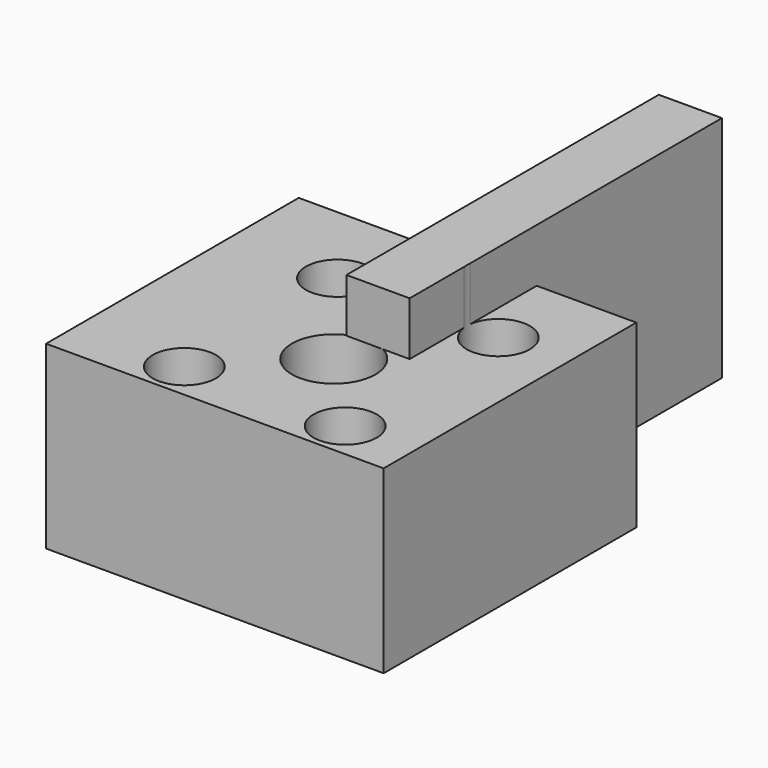
from build123d import *

# Parameters (mm, degrees)
F0_W     = 156.9848433137
F0_H     = 92.025604099
F1_DEPTH = 25.4
F2_W     = 135.7623711228
F2_H     = 72.5497286767
F4_DEPTH = 127
F6_D     = 25.4
F8_R     = 16.8146432666
F9_DEPTH = 72.5497286767


# Not quite as in the source:
# - a feature of the source that left no trace in its solid (it failed there, or was rolled back) is left out


with BuildPart() as f1:
    # F0 (on Right) → F1 (new body)
    with BuildSketch(Plane.YZ):
        with Locations((14.6216116846, 4.5173931867)):
            Rectangle(F0_W, F0_H)
    extrude(amount=F1_DEPTH)

    # F2 (on Front) → F4 (join)
    with BuildSketch(Plane.XZ):
        with Locations((-2.4367310107, -7.2724418715)):
            Rectangle(F2_W, F2_H)
    extrude(amount=F4_DEPTH)

    # F6 (through all)
    with Locations(Plane(origin=(0, 0, -43.5473062098), x_dir=(1, 0, 0), z_dir=(0, 0, -1))):
        with Locations((38.019452244, 112.0775043964), (38.019452244, 35.0753962994), (-26.6502853483, 35.0753962994), (-26.6502853483, 112.0775043964)):
            Hole(F6_D / 2)

    # F8 (on face) → F9 (cut, through all)
    with BuildSketch(Plane(origin=(0, 0, -43.5473062098), x_dir=(1, 0, 0), z_dir=(0, 0, -1))):
        with Locations((6.7373481579, 78.689865768)):
            Circle(F8_R)
    extrude(amount=-F9_DEPTH, mode=Mode.SUBTRACT)


solid = f1.part
